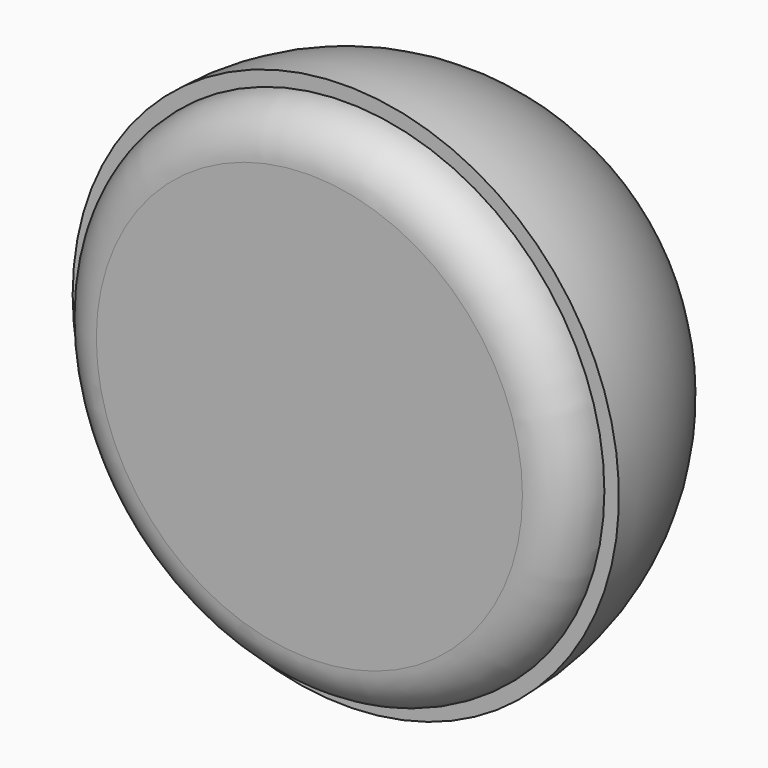
from build123d import *

# Parameters (mm, degrees)
F2_R     = 28.4
F3_DEPTH = 5
F4_R     = 4.99999


# Not quite as in the source:
# - a fillet or chamfer is up to 0.001 mm smaller than in the source, because OpenCascade refuses the exact size


with BuildPart() as f1:
    # F0 (on Top) → F1 (revolve)
    with BuildSketch(Plane.XY):
        with BuildLine():
            ThreePointArc((0, 37.1231260896), (-4.3133778971, 34.6519145578), (-4.3630481141, 29.6810345364))
            ThreePointArc((-4.3630481141, 29.6810345364), (-22.7034297346, 19.6100555402), (-30, 0))
            Line((-30, 0), (0, 0))
            Line((0, 0), (0, 27.1231260896))
            Line((0, 27.1231260896), (0, 30))
            Line((0, 30), (0, 37.1231260896))
        make_face()
    revolve(axis=Axis((0, 15, 0), (0, 1, 0)))

    # F2 (on Front) → F3 (join)
    with BuildSketch(Plane.XZ):
        Circle(F2_R)
    extrude(amount=F3_DEPTH)

    # F4 (radius 5 in the source; OpenCascade refuses exactly that, so slightly less here)
    f4_edges = [f1.edges().sort_by_distance(p)[0] for p in [
        (-28.4, -5, 0),
    ]]
    fillet(f4_edges, radius=F4_R)


solid = f1.part
